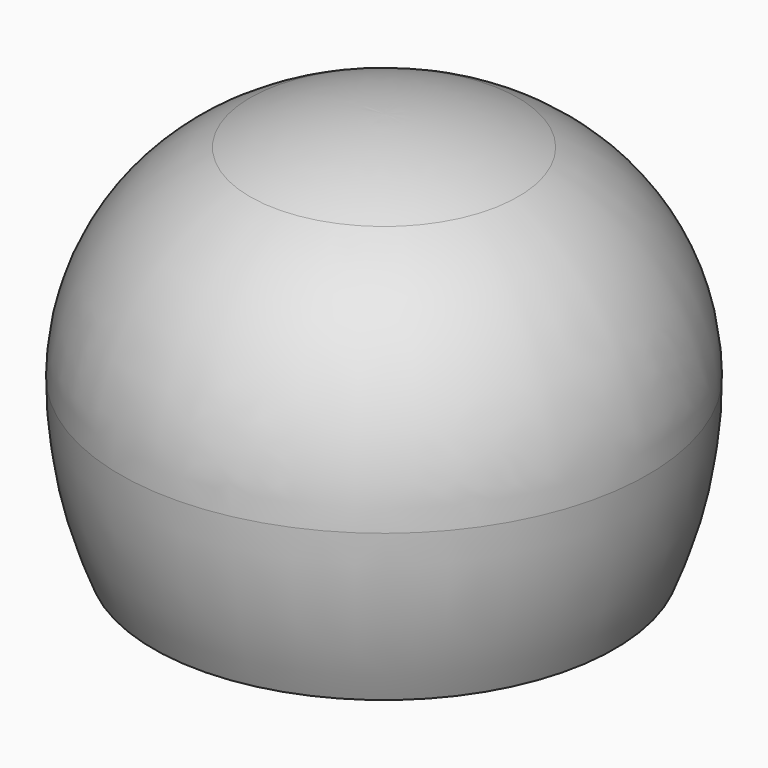
from build123d import *

# Parameters (mm, degrees)
F2_R = 1.2
F3_R = 1.5


# Not quite as in the source:
# - ends of sketch curves that miss each other by under 0.0002 mm in the source are joined


with BuildPart() as f1:
    # F0 (on Front) → F1 (revolve)
    with BuildSketch(Plane.XZ):
        with BuildLine():
            ThreePointArc((-3.15, 22.2222318008), (-3.903557352, 22.0716316829), (-4.65, 21.8890051469))
            Line((-4.65, 21.8890051469), (-4.65, 17.7222318008))
            Line((-4.65, 17.7222318008), (-3.15, 17.7222318008))
            Line((-3.15, 17.7222318008), (-3.15, 22.2222318008))
        make_face()
        with BuildLine():
            ThreePointArc((-7.4999988015, 20.8630687213), (-6.0966182517, 21.4360929938), (-4.65, 21.8890051469))
            ThreePointArc((-4.65, 21.8890051469), (-3.903557352, 22.0716316829), (-3.15, 22.2222318008))
            ThreePointArc((-3.15, 22.2222318008), (-1.5811115688, 22.430423481), (0, 22.5))
            Line((0, 22.5), (0, 24))
            ThreePointArc((0, 24), (-4.1581350796, 23.5515072433), (-8.1249988681, 22.2266581445))
            ThreePointArc((-8.1249988681, 22.2266581445), (-13.8619427254, 17.245190158), (-16, 9.9543562404))
            ThreePointArc((-16, 9.9543562404), (-15.4890851758, 4.8754171303), (-13.9768139545, 0))
            Line((-13.9768139545, 0), (-12.3382868923, 0))
            ThreePointArc((-12.3382868923, 0), (-13.9533457904, 4.8611693699), (-14.4999996005, 9.9543562404))
            ThreePointArc((-14.4999996005, 9.9543562404), (-12.5995043015, 16.4350973087), (-7.4999988015, 20.8630687213))
        make_face()
    revolve(axis=Axis((0, 0, 23.25), (0, 0, 1)))

    # F2
    f2_edges = [f1.edges().sort_by_distance(p)[0] for p in [
        (3.15, 0, 17.722232),
    ]]
    fillet(f2_edges, radius=F2_R)

    # F3
    f3_edges = [f1.edges().sort_by_distance(p)[0] for p in [
        (4.65, 0, 21.889005),
    ]]
    fillet(f3_edges, radius=F3_R)


solid = f1.part
